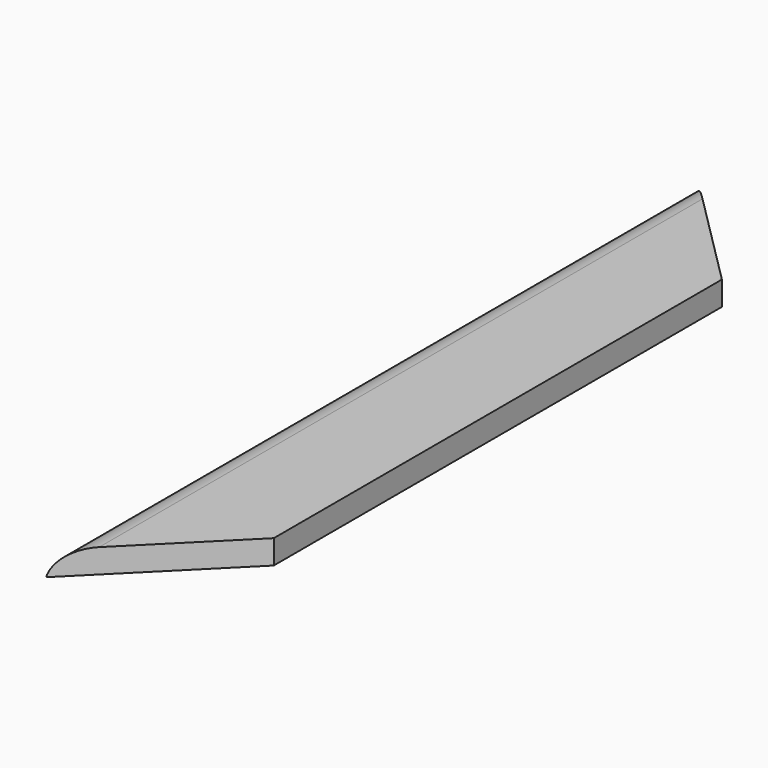
from build123d import *

# Parameters (mm, degrees)
F0_W        = 21
F0_H        = 135
F1_DEPTH    = 4
F3_DEPTH    = 4.001
F4_T1_DEPTH = 159.4948974279


# Not quite as in the source:
# - a fillet or chamfer that OpenCascade refuses, or shapes differently, is made with other operations: its cross-section is extruded or revolved along the edge and cut away or added


with BuildPart() as f1:
    # F0 (on Top) → F1 (new body)
    with BuildSketch(Plane.XY):
        Rectangle(F0_W, F0_H)
    extrude(amount=F1_DEPTH)

    # F2 (on face) → F3 (cut, through all)
    with BuildSketch(Plane.XY.offset(4)):
        Polygon((10.5, 67.5), (-10.5, 67.5), (10.5, 46.5), align=None)
        Polygon((10.5, -46.5), (-10.5, -67.5), (10.5, -67.5), align=None)
    extrude(amount=-F3_DEPTH, mode=Mode.SUBTRACT)

    # F4: fillet of radius 5 on 1 edges, made by hand

    # F4_s2 → F4_t1 (cut)
    with BuildSketch(Plane.XZ.offset(-79.7474487139)):
        with BuildLine():
            ThreePointArc((-5.6010205144, 4), (-8.7632981746, 2.8729833462), (-10.5, 0))
            Line((-10.5, 0), (-10.5, 4))
            Line((-10.5, 4), (-5.6010205144, 4))
        make_face()
    extrude(amount=F4_T1_DEPTH, mode=Mode.SUBTRACT)


solid = f1.part
